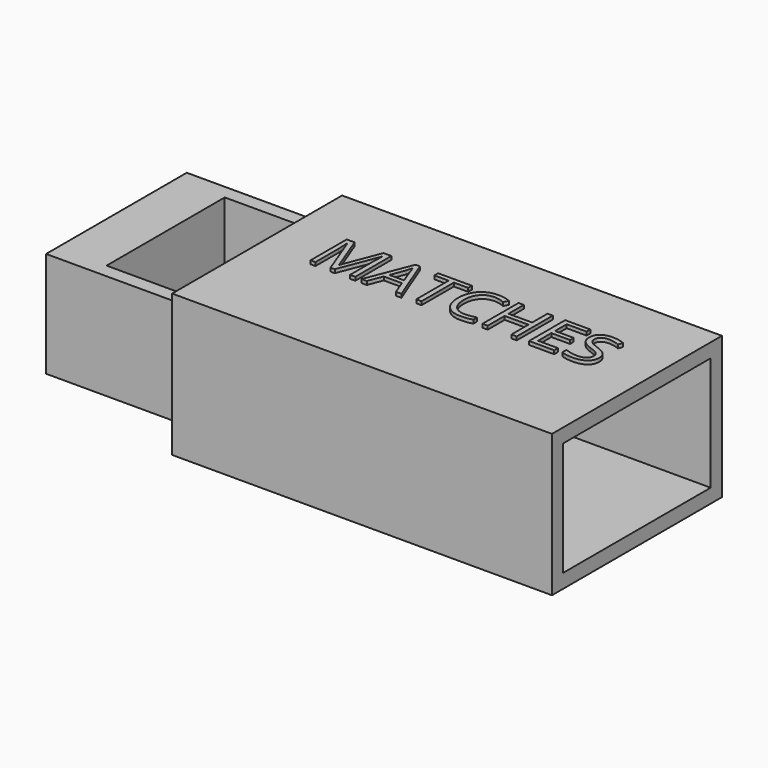
from build123d import *

# Parameters (mm, degrees)
F0_W         = 54
F0_H         = 25
F1_DEPTH     = 15
F2_W         = 50
F2_H         = 21
F3_DEPTH     = 13
F4_W         = 4
F4_H         = 4
F5_DEPTH     = 2.001
F6_W         = 30.2
F6_H         = 20.2
F6_W_2       = 26.2
F6_H_2       = 16.2
F7_DEPTH     = 54
F8_TEXT_SIZE = 8.982445191
F9_DEPTH     = 0.5
F11_DEPTH    = 5


# Not quite as in the source:
# - Text() gives the source's letters only with a copy of the font that has no kerning and outlines rounded to 1/6400 em; it was checked with that copy


with BuildPart() as f1:
    # F0 (on Top) → F1 (new body)
    with BuildSketch(Plane.XY):
        Rectangle(F0_W, F0_H)
    extrude(amount=F1_DEPTH)

    # F2 (on face) → F3 (cut)
    with BuildSketch(Plane.XY.offset(15)):
        Rectangle(F2_W, F2_H)
    extrude(amount=-F3_DEPTH, mode=Mode.SUBTRACT)

    # F4 (on face) → F5 (cut, through all)
    with BuildSketch(Plane.YZ.offset(-25)):
        with Locations((-8.5, 4)):
            Rectangle(F4_W, F4_H)
    extrude(amount=-F5_DEPTH, mode=Mode.SUBTRACT)

    # F11 (add): a face of the model
    f11_faces = [f1.faces().sort_by_distance(p)[0] for p in [
        (-25, 0.5291828794, 8.780155642),
    ]]
    extrude(f11_faces, amount=F11_DEPTH)


with BuildPart() as f7:
    # F6 (on face) → F7 (new body)
    with BuildSketch(Plane(origin=(-27, 0, 0), x_dir=(0, -1, 0), z_dir=(-1, 0, 0))):
        with Locations((0, 7.5)):
            Rectangle(F6_W, F6_H)
        with Locations((0, 7.5)):
            Rectangle(F6_W_2, F6_H_2, mode=Mode.SUBTRACT)
    extrude(amount=-F7_DEPTH)

    # F8 (on face) → F9 (join)
    with BuildSketch(Plane.XY.offset(17.6)):
        with Locations((-20.2764665116, 0)):
            Text('MATCHES', F8_TEXT_SIZE, font='Open Sans', text_align=(TextAlign.LEFT, TextAlign.BOTTOM))
    extrude(amount=F9_DEPTH)


with BuildPart() as f7_1:
    # F10: moved
    add(f7.part.moved(Location((20, 0, 0))))


solid = Compound([f1.part, f7_1.part])
